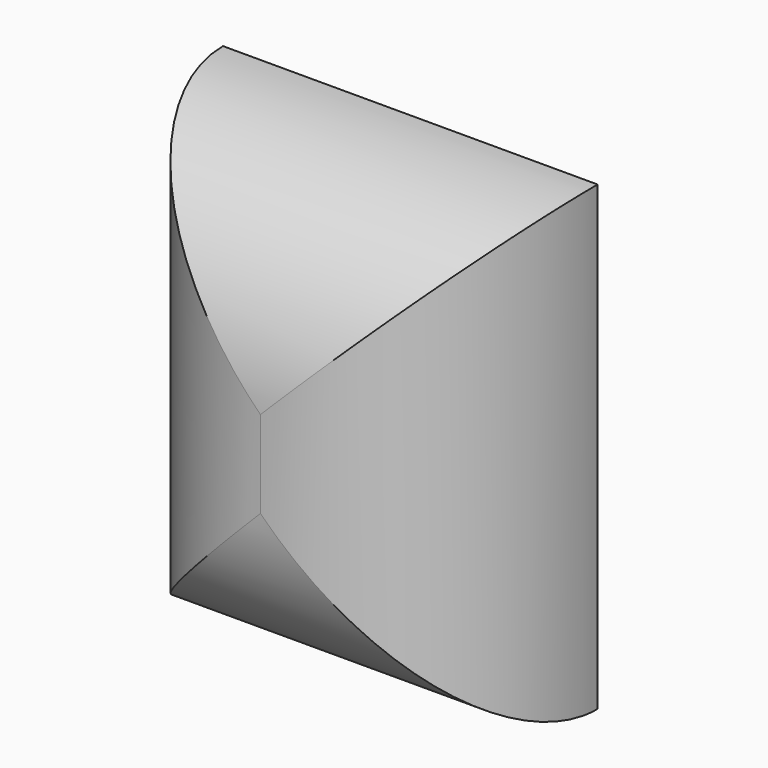
from build123d import *

# Parameters (mm, degrees)
F0_W     = 40
F0_H     = 25
F1_DEPTH = 49.3
F2_R     = 19.99999
F3_SIZE  = 5


# Not quite as in the source:
# - a fillet or chamfer is up to 0.001 mm smaller than in the source, because OpenCascade refuses the exact size


with BuildPart() as f1:
    # F0 (on Top) → F1 (new body)
    with BuildSketch(Plane.XY):
        with Locations((-24.3057886145, -13.9031428844)):
            Rectangle(F0_W, F0_H)
    extrude(amount=F1_DEPTH)

    # F2 (radius 20 in the source; OpenCascade refuses exactly that, so slightly less here)
    f2_edges = [f1.edges().sort_by_distance(p)[0] for p in [
        (-44.305789, -26.403143, 24.65),
        (-4.305789, -26.403143, 24.65),
        (-24.305789, -26.403143, 0),
        (-24.305789, -26.403143, 49.3),
    ]]
    fillet(f2_edges, radius=F2_R)

    # F3
    f3_edges = [f1.edges().sort_by_distance(p)[0] for p in [
        (-4.305789, -1.403143, 24.65),
        (-44.305789, -1.403143, 24.65),
        (-24.305789, -1.403143, 0),
        (-24.305789, -1.403143, 49.3),
    ]]
    chamfer(f3_edges, length=F3_SIZE)


solid = f1.part
